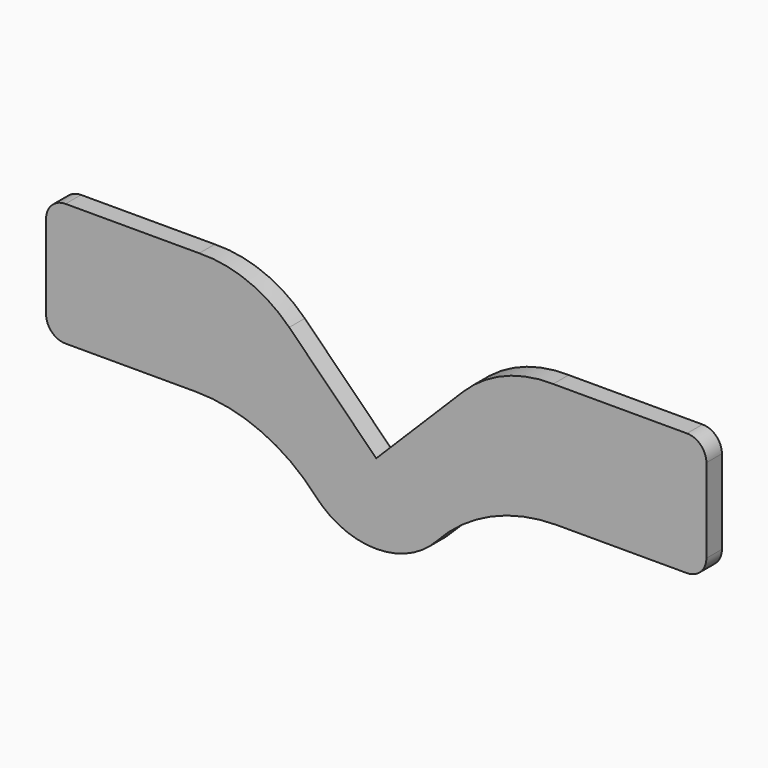
from build123d import *

# Parameters (mm, degrees)
F1_DEPTH = 3


# Not quite as in the source:
# - a feature of the source that left no trace in its solid (it failed there, or was rolled back) is left out


with BuildPart() as f1:
    # F0 (on Front) → F1 (new body)
    with BuildSketch(Plane.XZ):
        with BuildLine():
            ThreePointArc((-48, -22.5), (-50.1213203436, -23.3786796564), (-51, -25.5))
            Line((-51, -25.5), (-51, -38.5))
            ThreePointArc((-51, -38.5), (-50.1213203436, -40.6213203436), (-48, -41.5))
            Line((-48, -41.5), (-27.8693873068, -41.5))
            ThreePointArc((-27.8693873068, -41.5), (-17.7674216266, -43.6318936202), (-9.3883612413, -49.6639768483))
            ThreePointArc((-9.3883612413, -49.6639768483), (0, -53.8112770872), (9.3883612413, -49.6639768483))
            ThreePointArc((9.3883612413, -49.6639768483), (17.7674216266, -43.6318936202), (27.8693873068, -41.5))
            Line((27.8693873068, -41.5), (0, -41.5))
            Line((0, -41.5), (-13.4406096243, -28.0593903757))
            ThreePointArc((-13.4406096243, -28.0593903757), (-19.8179151952, -23.8538823154), (-27.3361149175, -22.5))
            Line((-27.3361149175, -22.5), (-48, -22.5))
        make_face()
        with BuildLine():
            Line((13.4406096243, -28.0593903757), (0, -41.5))
            Line((0, -41.5), (27.8693873068, -41.5))
            Line((27.8693873068, -41.5), (48, -41.5))
            ThreePointArc((48, -41.5), (50.1213203436, -40.6213203436), (51, -38.5))
            Line((51, -38.5), (51, -25.5))
            ThreePointArc((51, -25.5), (50.1213203436, -23.3786796564), (48, -22.5))
            Line((48, -22.5), (27.3361149175, -22.5))
            ThreePointArc((27.3361149175, -22.5), (19.8179151952, -23.8538823154), (13.4406096243, -28.0593903757))
        make_face()
    extrude(amount=F1_DEPTH)


solid = f1.part
